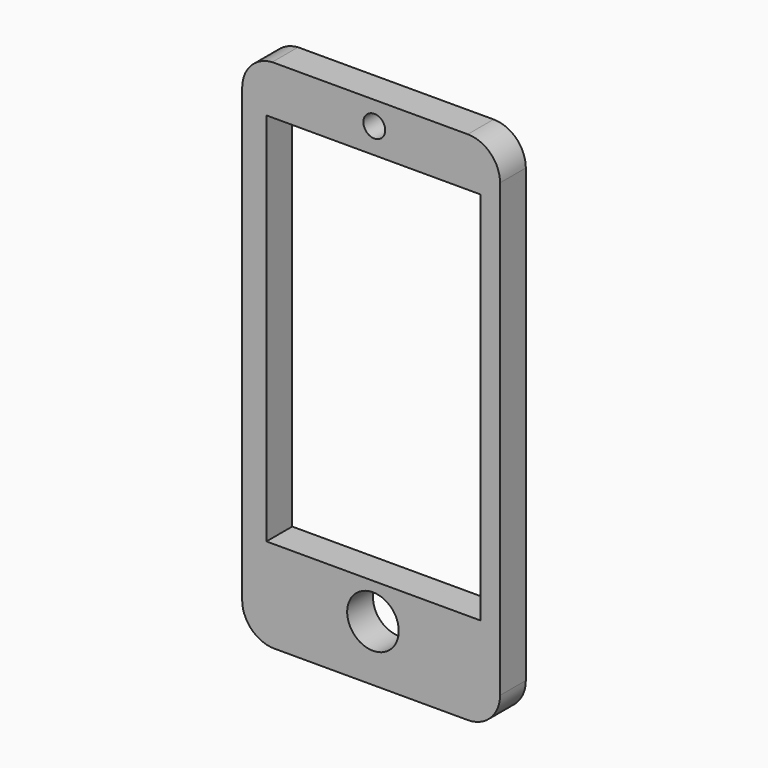
from build123d import *

# Parameters (mm, degrees)
F0_R     = 5.08
F0_R_2   = 0.0254
F0_W     = 42.184448801
F0_H     = 73.8955140114
F0_R_3   = 2.1477431595
F1_DEPTH = 6.35


# Not quite as in the source:
# - ends of sketch curves that miss each other by under 0.0002 mm in the source are joined


with BuildPart() as f1:
    # F0 (on Front) → F1 (new body)
    with BuildSketch(Plane.XZ):
        with BuildLine():
            ThreePointArc((-55.3989668916, 62.6738528225), (-59.6104772855, 60.6747009039), (-61.3217708439, 56.3382389188))
            Line((-61.3217708439, 56.3382389188), (-61.3217708439, -32.5617610812))
            ThreePointArc((-61.3217708439, -32.5617610812), (-59.4618989044, -37.0518891418), (-54.9717708439, -38.9117610812))
            Line((-54.9717708439, -38.9117610812), (-16.8717708439, -38.9117610812))
            ThreePointArc((-16.8717708439, -38.9117610812), (-12.3816427833, -37.0518891418), (-10.5217708439, -32.5617610812))
            Line((-10.5217708439, -32.5617610812), (-10.5217708439, 56.3382389188))
            ThreePointArc((-10.5217708439, 56.3382389188), (-12.3824811709, 60.8292052103), (-16.8741419405, 62.6882384761))
            Line((-16.8741419405, 62.6882384761), (-55.3989668916, 62.6738528225))
        make_face()
        with Locations((-35.5558670086, -27.8927588342)):
            Circle(F0_R, mode=Mode.SUBTRACT)
        with Locations((-46.6527380049, 56.3382389188)):
            Circle(F0_R_2, mode=Mode.SUBTRACT)
        with Locations((-35.4520422406, 16.1202251911)):
            Rectangle(F0_W, F0_H, mode=Mode.SUBTRACT)
        with Locations((-35.2948196232, 58.1041015685)):
            Circle(F0_R_3, mode=Mode.SUBTRACT)
    extrude(amount=F1_DEPTH)


solid = f1.part
